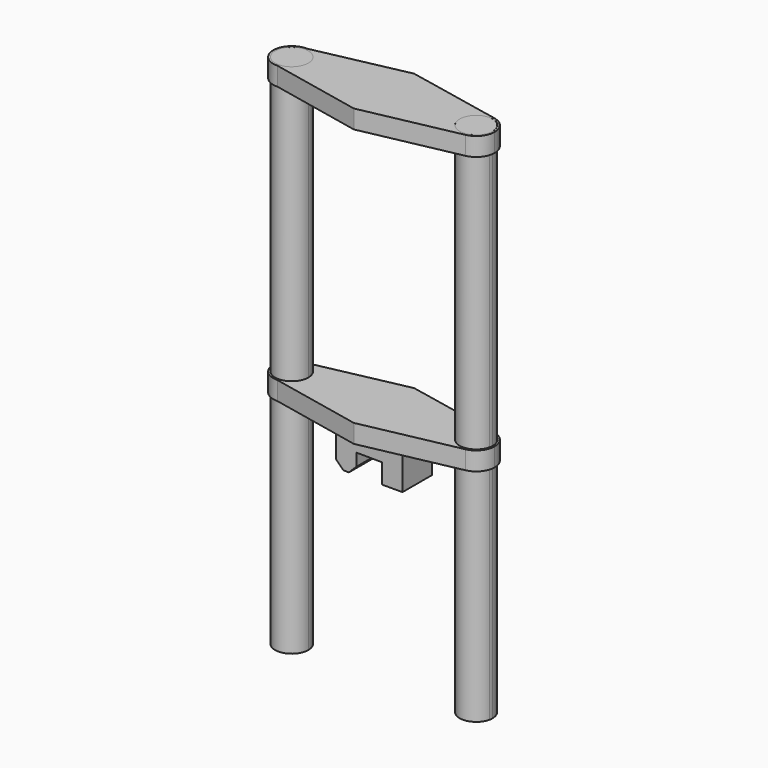
from build123d import *

# Parameters (mm, degrees)
F0_R     = 11.43
F1_DEPTH = 6.35
F6_DEPTH = 355.6
F8_DEPTH = 12.7
F9_SIZE  = 5.08


with BuildPart() as f1:
    # F0 (on Top) → F1 (new body, symmetric)
    with BuildSketch(Plane.XY):
        with BuildLine():
            ThreePointArc((76.1999999998, -0.000749004), (73.3389811571, 8.0294720257), (66.0449685374, 12.4416436575))
            ThreePointArc((66.0449685374, 12.4416436575), (50.7999999999, -0.0007858505), (66.0450407355, -12.4431268979))
            ThreePointArc((66.0450407355, -12.4431268979), (73.3390044552, -8.0309414879), (76.1999999998, -0.000749004))
        make_face()
        with Locations((63.4999999998, -0.000749004)):
            Circle(F0_R, mode=Mode.SUBTRACT)
        with BuildLine():
            ThreePointArc((-63.2525521899, -12.6975891248), (-54.4326799111, -8.8923397599), (-50.8, 0))
            ThreePointArc((-50.8, 0), (-54.4318821784, 8.8915262567), (-63.2502738856, 12.6975445212))
            ThreePointArc((-63.2502738856, 12.6975445212), (-76.1999999489, 0.0011393705), (-63.2525521899, -12.6975891248))
        make_face()
        with Locations((-63.5, 0)):
            Circle(F0_R, mode=Mode.SUBTRACT)
        with BuildLine():
            ThreePointArc((-63.2502738856, 12.6975445212), (-54.4318821784, 8.8915262567), (-50.8, 0))
            ThreePointArc((-50.8, 0), (-54.4326799111, -8.8923397599), (-63.2525521899, -12.6975891248))
            Line((-63.2525521899, -12.6975891248), (0, -25.9523869843))
            Line((0, -25.9523869843), (66.0450407355, -12.4431268979))
            ThreePointArc((66.0450407355, -12.4431268979), (50.7999999999, -0.0007858505), (66.0449685374, 12.4416436575))
            Line((66.0449685374, 12.4416436575), (0, 25.9504897099))
            Line((0, 25.9504897099), (-63.2502738856, 12.6975445212))
        make_face()
    extrude(amount=F1_DEPTH, both=True)


with BuildPart() as f2_1:
    # F2: copy of F1
    add(f1.part)


with BuildPart() as f4_1:
    # F4: copy of F1
    add(f1.part.moved(Location((0, 0, 190.5))))


with BuildPart() as f6:
    # F5 (on face) → F6 (new body)
    with BuildSketch(Plane.XY.offset(196.85)):
        with BuildLine():
            ThreePointArc((74.6565013441, -2.4861821162), (74.814113906, -1.3863449295), (74.8668094698, -0.2765220902))
            ThreePointArc((74.8668094698, -0.2765220902), (71.586586946, 7.8527431711), (63.5831147756, 11.4289488019))
            ThreePointArc((63.5831147756, 11.4289488019), (54.5562893746, -7.1179774149), (74.6565013441, -2.4861821162))
        make_face()
    extrude(amount=-F6_DEPTH)


with BuildPart() as f6b:
    # F5 (on face) → F6, piece 2 (new body)
    with BuildSketch(Plane.XY.offset(196.85)):
        with BuildLine():
            ThreePointArc((-52.07, 0), (-55.3299550342, 7.9934513982), (-63.2502738856, 11.4272716283))
            ThreePointArc((-63.2502738856, 11.4272716283), (-69.8260111671, 9.4792284929), (-74.1482627052, 4.1544435683))
            ThreePointArc((-74.1482627052, 4.1544435683), (-65.6136765694, -11.2328656789), (-52.07, 0))
        make_face()
    extrude(amount=-F6_DEPTH)


with BuildPart() as f8:
    # F7 (on Front) → F8 (new body, symmetric)
    with BuildSketch(Plane.XZ):
        Polygon((22.86, -33.5520400931), (22.86, -6.4680888293), (-22.86, -6.4680888293), (-22.86, -33.5520400931), (-8.89, -33.5520400931), (-8.89, -19.8643039912), (8.89, -20.0070151151), (8.89, -33.5520400931), align=None)
    extrude(amount=F8_DEPTH, both=True)

    # F9
    f9_edges = [f8.edges().sort_by_distance(p)[0] for p in [
        (-8.89, 0, -33.55204),
        (-22.86, 0, -33.55204),
    ]]
    chamfer(f9_edges, length=F9_SIZE)


solid = Compound([f1.part, f4_1.part, f6.part, f6b.part, f8.part])
